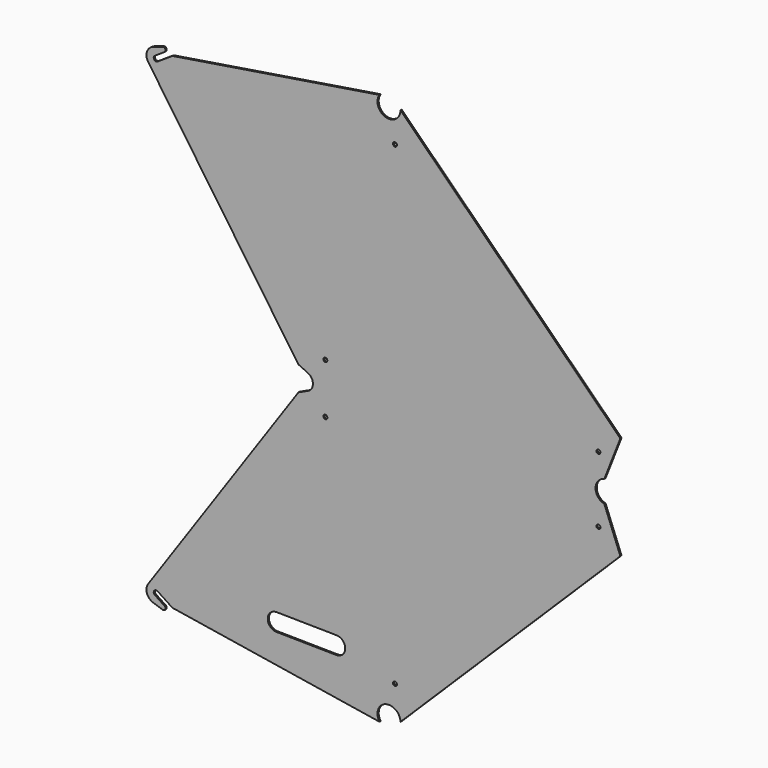
from build123d import *

# Parameters (mm, degrees)
F0_R     = 4
F1_DEPTH = 3
F5_DEPTH = 3
F8_DEPTH = 25
F9_DEPTH = 25


# Not quite as in the source:
# - ends of sketch curves that miss each other by under 0.0002 mm in the source are joined


with BuildPart() as f1:
    # F0 (on Front) → F1 (new body)
    with BuildSketch(Plane.XZ):
        with BuildLine():
            ThreePointArc((585.5387718609, -70.1653972109), (584.1001986375, -63.1555680907), (591.1100276795, -61.716994486))
            Line((591.1100276795, -61.716994486), (620.6688569888, -81.2094156242))
            Line((620.6688569888, -81.2094156242), (1035.0006136748, -147.2807863546))
            ThreePointArc((1035.0006136748, -147.2807863546), (1046.8897667562, -112.3036113444), (1076.917388022, -133.8232928895))
            Line((1076.917388022, -133.8232928895), (1516.7807656982, 301.1320483365))
            Line((1516.7807656982, 301.1320483365), (1482.3585617346, 388.849064))
            Line((1482.3585617346, 388.849064), (878.7694007197, 388.849064))
            Line((878.7694007197, 388.849064), (572.7458963991, -54.0303683051))
            ThreePointArc((572.7458963991, -54.0303683051), (569.563169725, -71.6485447179), (582.0179839674, -84.5096290961))
            Line((582.0179839674, -84.5096290961), (601.192342, -91.021836))
            ThreePointArc((601.192342, -91.021836), (606.4892645676, -88.6748164062), (605.0838007766, -83.0542683087))
            Line((605.0838007766, -83.0542683087), (585.5387718609, -70.1653972109))
        make_face()
        with Locations((1065.920517, -70.202665)):
            Circle(F0_R, mode=Mode.SUBTRACT)
        with Locations((926.6393642448, 354.4944504476)):
            Circle(F0_R, mode=Mode.SUBTRACT)
        with Locations((1472.9055166245, 338.570445776)):
            Circle(F0_R, mode=Mode.SUBTRACT)
    extrude(amount=F1_DEPTH)


with BuildPart() as f3_1:
    # F3: instance of F1
    add(f1.part.mirror(Plane(origin=(1180.5639812271, -1.5, 404.749064), x_dir=(1, 0, 0), z_dir=(0, 0, 1))))


with BuildPart() as f1_1:
    add(f1.part)

    add(f3_1.part)  # F5 merges F3_1
    # F4 (on face) → F5 (join, through all)
    with BuildSketch(Plane.XZ.offset(3)):
        with BuildLine():
            ThreePointArc((1473.8185102428, 388.849064), (1467.2383092365, 404.749064), (1473.8185102428, 420.649064))
            Line((1473.8185102428, 420.649064), (891.5892198284, 420.649064))
            ThreePointArc((891.5892198284, 420.649064), (901.7789530754, 404.749064), (891.5892198284, 388.849064))
            Line((891.5892198284, 388.849064), (1473.8185102428, 388.849064))
        make_face()
    extrude(amount=-F5_DEPTH)

    # F7 (on face) → F8 (cut)
    with BuildSketch(Plane.XZ.offset(3)):
        with BuildLine():
            Line((949.1413939246, -22.7795250632), (829.1413939246, -21.0615598373))
            ThreePointArc((829.1413939246, -21.0615598373), (811.3926761125, -38.3092558002), (828.6403720754, -56.0579736122))
            Line((828.6403720754, -56.0579736122), (948.6403720754, -57.7759388381))
            ThreePointArc((948.6403720754, -57.7759388381), (966.3890898875, -40.5282428752), (949.1413939246, -22.7795250632))
        make_face()
    extrude(amount=-F8_DEPTH, mode=Mode.SUBTRACT)

    # F6 (on face) → F9 (cut)
    with BuildSketch(Plane.XZ.offset(3)):
        with BuildLine():
            ThreePointArc((891.5892198284, 388.849064), (901.7789530754, 404.749064), (891.5892198284, 420.649064))
            Line((891.5892198284, 420.649064), (872.8003346685, 429.2875396296))
            Line((872.8003346685, 429.2875396296), (872.8003346685, 380.2105883704))
            Line((872.8003346685, 380.2105883704), (891.5892198284, 388.849064))
        make_face()
        with BuildLine():
            Line((1484.726747317, 382.814291443), (1484.726747317, 426.683836557))
            ThreePointArc((1484.726747317, 426.683836557), (1467.2383092365, 404.749064), (1484.726747317, 382.814291443))
        make_face()
    extrude(amount=-F9_DEPTH, mode=Mode.SUBTRACT)


solid = f1_1.part
